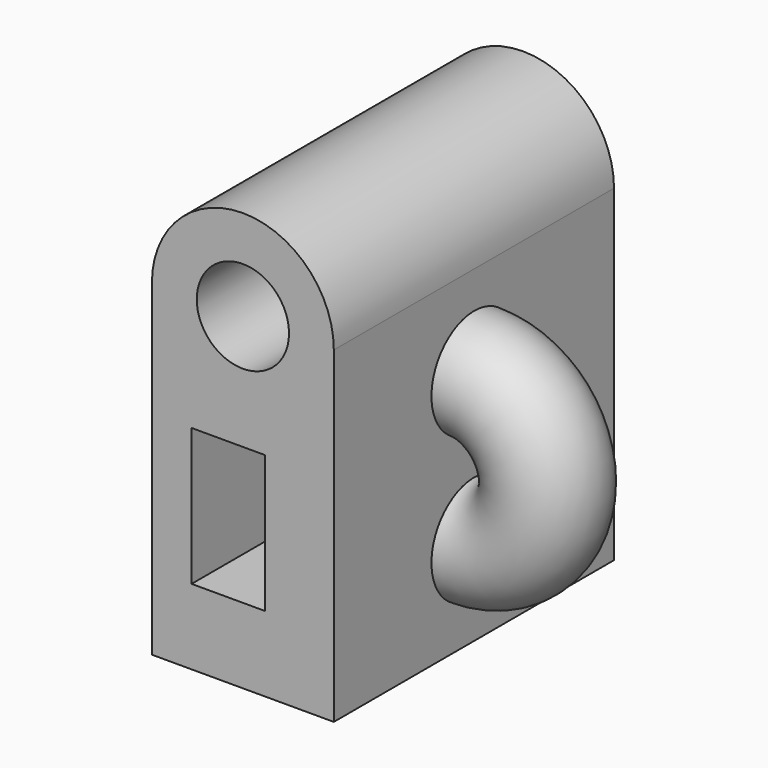
from build123d import *

# Parameters (mm, degrees)
F0_R     = 8.3642663508
F1_DEPTH = 63.5
F2_W     = 13.291940093
F2_H     = 24.8854812235
F3_DEPTH = 25.4
F4_R     = 9.7063550573
F5_ANGLE = 180


# Not quite as in the source:
# - a feature names something its author has since deleted; it is built from what else it names


with BuildPart() as f1:
    # F0 (on Front) → F1 (new body)
    with BuildSketch(Plane.XZ):
        with BuildLine():
            Line((-16.4914578199, -29.6862870455), (16.4914578199, -29.6862870455))
            Line((16.4914578199, -29.6862870455), (16.4914578199, 29.6862870455))
            ThreePointArc((16.4914578199, 29.6862870455), (0, 46.1777448654), (-16.4914578199, 29.6862870455))
            Line((-16.4914578199, 29.6862870455), (-16.4914578199, -29.6862870455))
        make_face()
        with Locations((0, 29.6862870455)):
            Circle(F0_R, mode=Mode.SUBTRACT)
    extrude(amount=F1_DEPTH)

    # F2 (on face) → F3 (cut)
    with BuildSketch(Plane.XZ.offset(63.5)):
        with Locations((-2.6479512453, -3.5954387859)):
            Rectangle(F2_W, F2_H)
    extrude(amount=-F3_DEPTH, mode=Mode.SUBTRACT)

    # F4 (on face) → F5 (revolve)
    with BuildSketch(Plane.YZ.offset(16.4914578199)):
        with Locations((-31.6691994667, 13.287819922)):
            Circle(F4_R)
    revolve(axis=Axis((16.4914578199, -31.75, 0), (0, 1, 0)), revolution_arc=F5_ANGLE)


solid = f1.part
